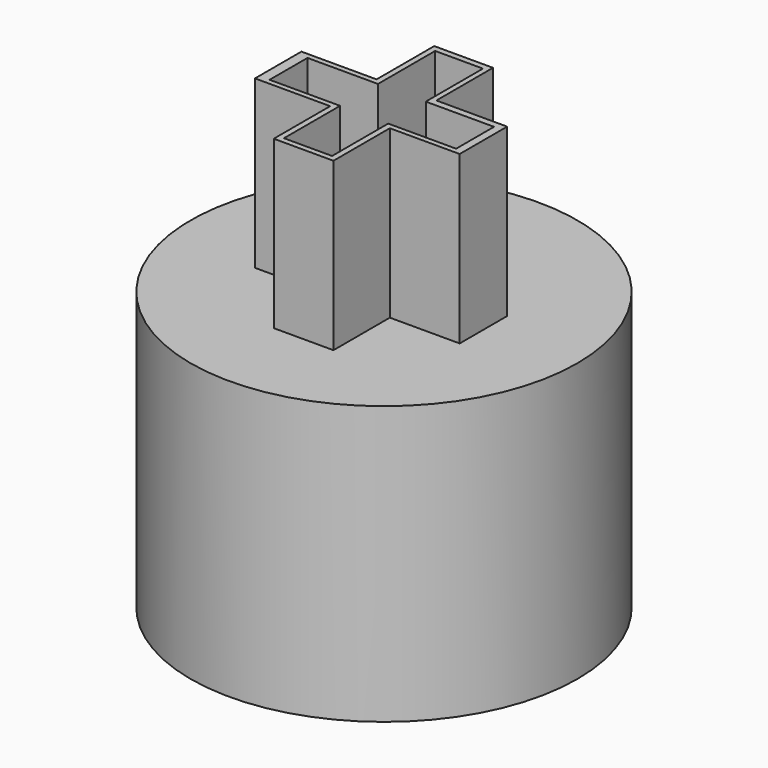
from build123d import *

# Parameters (mm, degrees)
F1_DEPTH     = 3.6
F2_R         = 4.1756906524
F3_DEPTH     = 6
F4_TEXT_SIZE = 5.2951784002
F5_DEPTH     = 0.5


# Not quite as in the source:
# - Text() gives the source's letters only with a copy of the font that has no kerning and outlines rounded to 1/6400 em; it was checked with that copy


with BuildPart() as f1:
    # F0 (on Top) → F1 (new body)
    with BuildSketch(Plane.XY):
        Polygon((-7.7989660203, 3.5650415812), (-7.7989660203, 3.4051602706), (-7.7989660203, 2.0434679464), (-6.5105301328, 2.0434679464), (-6.5105301328, 3.5650415812), (-5.0030690618, 3.5650415812), (-5.0030690618, 4.8457924277), (-6.5304460004, 4.8457924277), (-6.5304460004, 6.3735153526), (-7.7989660203, 6.3735153526), (-7.7989660203, 4.8178280704), (-9.4217183068, 4.8178280704), (-9.4217183068, 3.5650415812), align=None)
        Polygon((-7.6761739329, 4.7018225305), (-7.6761739329, 6.222656928), (-7.6761739329, 6.2444242649), (-6.6442829557, 6.2444242649), (-6.6442829557, 4.7018225305), (-5.1710316911, 4.7018225305), (-5.1710316911, 3.6793935578), (-6.6377311014, 3.6793935578), (-6.6377311014, 2.1653522272), (-7.6761739329, 2.1653522272), (-7.6761739329, 3.6793935578), (-9.1974688694, 3.6793935578), (-9.1974688694, 4.7018225305), align=None, mode=Mode.SUBTRACT)
    extrude(amount=F1_DEPTH)

    # F2 (on face) → F3 (join)
    with BuildSketch(Plane(origin=(0, 0, 0), x_dir=(1, 0, 0), z_dir=(0, 0, -1))):
        with Locations((-7.1774572134, -4.2408960871)):
            Circle(F2_R)
    extrude(amount=F3_DEPTH)

    # F4 (on face) → F5 (join)
    with BuildSketch(Plane(origin=(0, 0, -6), x_dir=(1, 0, 0), z_dir=(0, 0, -1))):
        with Locations((-8.8503714651, -6.2839202583)):
            Text('>', F4_TEXT_SIZE, font='Open Sans', text_align=(TextAlign.LEFT, TextAlign.BOTTOM))
    extrude(amount=-F5_DEPTH)


solid = f1.part
